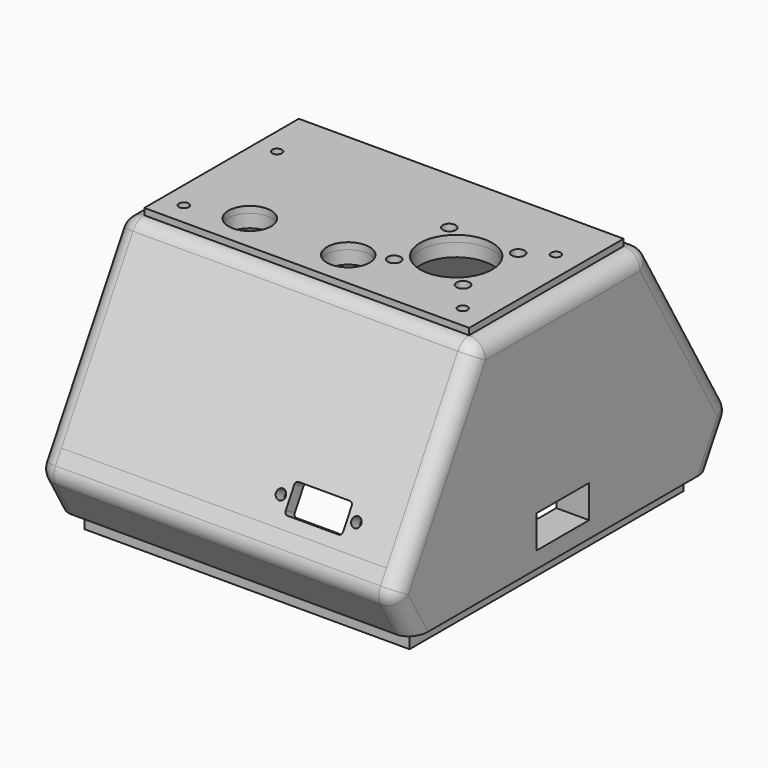
from build123d import *

# Parameters (mm, degrees)
F0_W          = 100
F0_H          = 60
F0_R          = 1.5
F0_R_2        = 6.5
F0_R_3        = 2
F0_R_4        = 11
F1_DEPTH      = 4
F2_R          = 2.5
F2_R_2        = 1.5
F3_DEPTH      = 35
F4_R          = 2.5
F4_R_2        = 1.5
F5_DEPTH      = 25
F6_W          = 2
F6_H          = 4
F7_DEPTH      = 100
F9_DEPTH      = 5
F10_W         = 30.2208131179
F10_H         = 20
F11_DEPTH     = 4
F13_DEPTH     = 109
F14_W         = 99
F14_H         = 104.2820323028
F15_DEPTH     = 6
F16_T1_DEPTH  = 58.8897274573
F16_T3_DEPTH  = 99
F16_T5_DEPTH  = 58.8452994616
F16_T7_DEPTH  = 24.6132486541
F16_T9_DEPTH  = 58.8897274573
F16_T11_DEPTH = 74.2764788033
F16_T13_DEPTH = 111.2168783649
F16_T15_DEPTH = 24.6132486541
F16_T17_DEPTH = 58.8897274573
F16_T22_DEPTH = 5
F16_T28_DEPTH = 5
F16_T34_DEPTH = 5
F16_T40_DEPTH = 5
F16_T46_DEPTH = 5
F16_T52_DEPTH = 5
F16_T58_DEPTH = 5
F17_W         = 89
F17_H         = 94.2820323028
F18_DEPTH     = 25
F19_W         = 20
F19_H         = 10
F20_DEPTH     = 10
F21_W         = 2
F21_H         = 2.6410161514
F21_W_2       = 3
F21_H_2       = 0.3589838486
F22_DEPTH     = 15
F23_R         = 1.25
F24_DEPTH     = 10
F25_R         = 0.99999
F26_W         = 17.5
F26_H         = 8.5
F26_R         = 1.5
F27_DEPTH     = 25
F28_R         = 1
F29_W         = 99
F29_H         = 58.8452994616
F29_R         = 1.5
F29_R_2       = 6.5
F29_R_3       = 2
F29_R_4       = 11
F30_DEPTH     = 2
F31_DEPTH     = 50


# Not quite as in the source:
# - a fillet or chamfer that OpenCascade refuses, or shapes differently, is made with other operations: its cross-section is extruded or revolved along the edge and cut away or added
# - a fillet or chamfer is up to 0.001 mm smaller than in the source, because OpenCascade refuses the exact size
# - a feature names something its author has since deleted; it is built from what else it names


with BuildPart() as f1:
    # F0 (on Top) → F1 (new body)
    with BuildSketch(Plane.XY):
        Rectangle(F0_W, F0_H)
        with Locations((-42.5, -22.5)):
            Circle(F0_R, mode=Mode.SUBTRACT)
        with Locations((-26, -18)):
            Circle(F0_R_2, mode=Mode.SUBTRACT)
        with Locations((4, -18)):
            Circle(F0_R_2, mode=Mode.SUBTRACT)
        with Locations((42.5, -22.5)):
            Circle(F0_R, mode=Mode.SUBTRACT)
        with Locations((14, -13)):
            Circle(F0_R_3, mode=Mode.SUBTRACT)
        with Locations((24.5, -2.5)):
            Circle(F0_R_4, mode=Mode.SUBTRACT)
        with Locations((35, -13)):
            Circle(F0_R_3, mode=Mode.SUBTRACT)
        with Locations((-42.5, 13)):
            Circle(F0_R, mode=Mode.SUBTRACT)
        with Locations((14, 8)):
            Circle(F0_R_3, mode=Mode.SUBTRACT)
        with Locations((35, 8)):
            Circle(F0_R_3, mode=Mode.SUBTRACT)
        with Locations((42.5, 13)):
            Circle(F0_R, mode=Mode.SUBTRACT)
    extrude(amount=F1_DEPTH)

    # F2 (on face) → F3 (join)
    with BuildSketch(Plane(origin=(0, 0, 0), x_dir=(1, 0, 0), z_dir=(0, 0, -1))):
        with Locations((-42.5, 22.5)):
            Circle(F2_R)
        with Locations((-42.5, 22.5)):
            Circle(F2_R_2, mode=Mode.SUBTRACT)
        with Locations((-42.5, -13)):
            Circle(F2_R)
        with Locations((-42.5, -13)):
            Circle(F2_R_2, mode=Mode.SUBTRACT)
        with Locations((42.5, -13)):
            Circle(F2_R)
        with Locations((42.5, -13)):
            Circle(F2_R_2, mode=Mode.SUBTRACT)
        with Locations((42.5, 22.5)):
            Circle(F2_R)
        with Locations((42.5, 22.5)):
            Circle(F2_R_2, mode=Mode.SUBTRACT)
    extrude(amount=F3_DEPTH)

    # F4 (on face) → F5 (join)
    with BuildSketch(Plane.XY.offset(4)):
        with Locations((-42.5, 13)):
            Circle(F4_R)
        with Locations((-42.5, 13)):
            Circle(F4_R_2, mode=Mode.SUBTRACT)
        with Locations((42.5, 13)):
            Circle(F4_R_2)
        with Locations((42.5, -22.5)):
            Circle(F4_R_2)
        with Locations((-42.5, -22.5)):
            Circle(F4_R)
        with Locations((-42.5, -22.5)):
            Circle(F4_R_2, mode=Mode.SUBTRACT)
    extrude(amount=-F5_DEPTH)

    # F6 (on face) → F7 (join)
    with BuildSketch(Plane.YZ.offset(50)):
        with Locations((-29, 2)):
            Rectangle(F6_W, F6_H)
        Polygon((-57.5, -47.6313972081), (-30, 0), (-30, 4), (-32.3094010768, 4), (-33.4641016151, 2), (-60.9641016151, -45.6313972081), (-64.6410161514, -52), (-60.0222139979, -52), align=None)
        with Locations((29, 2)):
            Rectangle(F6_W, F6_H)
        Polygon((30, 4), (30, 0), (57.5, -47.6313972081), (60.0222139979, -52), (64.6410161514, -52), (60.9641016151, -45.6313972081), (33.4641016151, 2), (32.3094010768, 4), align=None)
    extrude(amount=-F7_DEPTH)

    # F8 (on face) → F9 (join)
    with BuildSketch(Plane.YZ.offset(50)):
        Polygon((-32.3094010768, 4), (-64.6410161514, -52), (64.6410161514, -52), (32.3094010768, 4), align=None)
    extrude(amount=F9_DEPTH)

    # F10 (on face) → F11 (join)
    with BuildSketch(Plane(origin=(-50, 0, 0), x_dir=(0, -1, 0), z_dir=(-1, 0, 0))):
        Polygon((-32.3094010768, 4), (-64.6410161514, -52), (64.6410161514, -52), (32.3094010768, 4), align=None)
        with Locations((4.7969543375, -25.0177697837)):
            Rectangle(F10_W, F10_H, mode=Mode.SUBTRACT)
    extrude(amount=F11_DEPTH)

    # F12 (on face) → F13 (join, through all)
    with BuildSketch(Plane(origin=(-54, 0, 0), x_dir=(0, -1, 0), z_dir=(-1, 0, 0))):
        Polygon((-63.0000010133, -52), (-64.6410161514, -52), (-57.1410161514, -64.9903810568), (57.1410161514, -64.9903810568), (64.6410161514, -52), align=None)
    extrude(amount=-F13_DEPTH)

    # F14 (on face) → F15 (join)
    with BuildSketch(Plane(origin=(0, 0, -64.9903810568), x_dir=(1, 0, 0), z_dir=(0, 0, -1))):
        with Locations((0.5, 0)):
            Rectangle(F14_W, F14_H)
    extrude(amount=F15_DEPTH)

    # F16: fillet of radius 5 on 13 edges, made by hand

    # F16_s2 → F16_t1 (cut)
    with BuildSketch(Plane(origin=(0, -37.2335388633, -64.4903810568), x_dir=(1, 0, 0), z_dir=(0, 0.5, 0.8660254038))):
        with BuildLine():
            ThreePointArc((-54, -24.9807621135), (-52.5355339059, -28.5162960195), (-49, -29.9807621135))
            Line((-49, -29.9807621135), (-54, -29.9807621135))
            Line((-54, -29.9807621135), (-54, -24.9807621135))
        make_face()
    extrude(amount=F16_T1_DEPTH, mode=Mode.SUBTRACT)

    # F16_s4 → F16_t3 (cut)
    with BuildSketch(Plane.YZ.offset(-49)):
        with BuildLine():
            ThreePointArc((-29.4226497308, 4), (-31.9226497308, 3.3301270189), (-33.7527767497, 1.5))
            Line((-33.7527767497, 1.5), (-32.3094010768, 4))
            Line((-32.3094010768, 4), (-29.4226497308, 4))
        make_face()
        with BuildLine():
            ThreePointArc((-63.1976404784, -49.5), (-63.8675134595, -52), (-63.1976404784, -54.5))
            Line((-63.1976404784, -54.5), (-64.6410161514, -52))
            Line((-64.6410161514, -52), (-63.1976404784, -49.5))
        make_face()
        with BuildLine():
            ThreePointArc((29.4226497308, 4), (31.9226497308, 3.3301270189), (33.7527767497, 1.5))
            Line((33.7527767497, 1.5), (32.3094010768, 4))
            Line((32.3094010768, 4), (29.4226497308, 4))
        make_face()
    extrude(amount=F16_T3_DEPTH, mode=Mode.SUBTRACT)

    # F16_s6 → F16_t5 (cut)
    with BuildSketch(Plane.XZ.offset(-29.4226497308)):
        with BuildLine():
            ThreePointArc((-49, 4), (-52.5355339059, 2.5355339059), (-54, -1))
            Line((-54, -1), (-54, 4))
            Line((-54, 4), (-49, 4))
        make_face()
        with BuildLine():
            ThreePointArc((50, 4), (53.5355339059, 2.5355339059), (55, -1))
            Line((55, -1), (55, 4))
            Line((55, 4), (50, 4))
        make_face()
    extrude(amount=F16_T5_DEPTH, mode=Mode.SUBTRACT)

    # F16_s8 → F16_t7 (cut)
    with BuildSketch(Plane(origin=(0, 20.1064064606, -34.8253175473), x_dir=(1, 0, 0), z_dir=(0, -0.5, 0.8660254038))):
        with BuildLine():
            ThreePointArc((-54, -76.9807621135), (-52.5355339059, -80.5162960195), (-49, -81.9807621135))
            Line((-49, -81.9807621135), (-54, -81.9807621135))
            Line((-54, -81.9807621135), (-54, -76.9807621135))
        make_face()
        with BuildLine():
            ThreePointArc((55, -76.9807621135), (53.5355339059, -80.5162960195), (50, -81.9807621135))
            Line((50, -81.9807621135), (55, -81.9807621135))
            Line((55, -81.9807621135), (55, -76.9807621135))
        make_face()
    extrude(amount=F16_T7_DEPTH, mode=Mode.SUBTRACT)

    # F16_s10 → F16_t9 (cut)
    with BuildSketch(Plane(origin=(0, -7.7886751346, -13.4903810568), x_dir=(1, 0, 0), z_dir=(0, -0.5, -0.8660254038))):
        with BuildLine():
            ThreePointArc((50, 29.9807621135), (53.5355339059, 28.5162960195), (55, 24.9807621135))
            Line((55, 24.9807621135), (55, 29.9807621135))
            Line((55, 29.9807621135), (50, 29.9807621135))
        make_face()
    extrude(amount=F16_T9_DEPTH, mode=Mode.SUBTRACT)

    # F16_s12 → F16_t11 (cut)
    with BuildSketch(Plane(origin=(0, 7.7886751346, -13.4903810568), x_dir=(1, 0, 0), z_dir=(0, 0.5, -0.8660254038))):
        with BuildLine():
            ThreePointArc((-54, -24.9807621135), (-52.5355339059, -28.5162960195), (-49, -29.9807621135))
            Line((-49, -29.9807621135), (-54, -29.9807621135))
            Line((-54, -29.9807621135), (-54, -24.9807621135))
        make_face()
    extrude(amount=F16_T11_DEPTH, mode=Mode.SUBTRACT)

    # F16_s14 → F16_t13 (cut)
    with BuildSketch(Plane.YZ.offset(-61.2168783649)):
        with BuildLine():
            ThreePointArc((63.1976404784, -49.5), (63.8675134595, -52), (63.1976404784, -54.5))
            Line((63.1976404784, -54.5), (64.6410161514, -52))
            Line((64.6410161514, -52), (63.1976404784, -49.5))
        make_face()
    extrude(amount=F16_T13_DEPTH, mode=Mode.SUBTRACT)

    # F16_s16 → F16_t15 (cut)
    with BuildSketch(Plane(origin=(0, -7.7997821335, -13.5096189432), x_dir=(1, 0, 0), z_dir=(0, -0.5, -0.8660254038))):
        with BuildLine():
            ThreePointArc((55, -76.9807621135), (53.5355339059, -80.5162960195), (50, -81.9807621135))
            Line((50, -81.9807621135), (55, -81.9807621135))
            Line((55, -81.9807621135), (55, -76.9807621135))
        make_face()
    extrude(amount=F16_T15_DEPTH, mode=Mode.SUBTRACT)

    # F16_s18 → F16_t17 (cut)
    with BuildSketch(Plane(origin=(0, 37.2335388633, -64.4903810568), x_dir=(1, 0, 0), z_dir=(0, -0.5, 0.8660254038))):
        with BuildLine():
            ThreePointArc((50, 29.9807621135), (53.5355339059, 28.5162960195), (55, 24.9807621135))
            Line((55, 24.9807621135), (55, 29.9807621135))
            Line((55, 29.9807621135), (50, 29.9807621135))
        make_face()
    extrude(amount=F16_T17_DEPTH, mode=Mode.SUBTRACT)


with BuildPart() as f16_tool20:
    # F16_s21 → F16_t22 (new body)
    with BuildSketch(Plane.YZ.offset(-49)):
        Polygon((-58.8675134595, -52), (-63.1976404784, -54.5), (-64.6410161514, -52), (-63.1976404784, -49.5), align=None)
    extrude(amount=-F16_T22_DEPTH)

    # F16_s23 → F16_t24 (revolve, cut)
    with BuildSketch(Plane(origin=(-49, -58.8675134595, -52), x_dir=(0, 1, 0), z_dir=(0, 0, 1))):
        with BuildLine():
            ThreePointArc((0, -5), (5, 0), (0, 5))
            Line((0, 5), (0, -5))
        make_face()
    revolve(axis=Axis((-49, -58.8675134595, -52), (-1, 0, 0)), mode=Mode.SUBTRACT)


with BuildPart() as f1_1:
    add(f1.part)

    # F16_t19: cut F16_tool20
    add(f16_tool20.part, mode=Mode.SUBTRACT)


with BuildPart() as f16_tool26:
    # F16_s27 → F16_t28 (new body)
    with BuildSketch(Plane.YZ.offset(-49)):
        Polygon((-29.4226497308, -1), (-33.7527767497, 1.5), (-32.3094010768, 4), (-29.4226497308, 4), align=None)
    extrude(amount=-F16_T28_DEPTH)

    # F16_s29 → F16_t30 (revolve, cut)
    with BuildSketch(Plane(origin=(-49, -29.4226497308, -1), x_dir=(0, 0.5, -0.8660254038), z_dir=(0, 0.8660254038, 0.5))):
        with BuildLine():
            ThreePointArc((0, -5), (5, 0), (0, 5))
            Line((0, 5), (0, -5))
        make_face()
    revolve(axis=Axis((-49, -29.4226497308, -1), (-1, 0, 0)), mode=Mode.SUBTRACT)


with BuildPart() as f1_2:
    add(f1_1.part)

    # F16_t25: cut F16_tool26
    add(f16_tool26.part, mode=Mode.SUBTRACT)


with BuildPart() as f16_tool32:
    # F16_s33 → F16_t34 (new body)
    with BuildSketch(Plane.YZ.offset(50)):
        Polygon((-29.4226497308, -1), (-33.7527767497, 1.5), (-32.3094010768, 4), (-29.4226497308, 4), align=None)
    extrude(amount=F16_T34_DEPTH)

    # F16_s35 → F16_t36 (revolve, cut)
    with BuildSketch(Plane(origin=(50, -29.4226497308, -1), x_dir=(0, 0.5, -0.8660254038), z_dir=(0, -0.8660254038, -0.5))):
        with BuildLine():
            ThreePointArc((0, -5), (5, 0), (0, 5))
            Line((0, 5), (0, -5))
        make_face()
    revolve(axis=Axis((50, -29.4226497308, -1), (1, 0, 0)), mode=Mode.SUBTRACT)


with BuildPart() as f1_3:
    add(f1_2.part)

    # F16_t31: cut F16_tool32
    add(f16_tool32.part, mode=Mode.SUBTRACT)


with BuildPart() as f16_tool38:
    # F16_s39 → F16_t40 (new body)
    with BuildSketch(Plane.YZ.offset(-49)):
        Polygon((29.4226497308, -1), (33.7527767497, 1.5), (32.3094010768, 4), (29.4226497308, 4), align=None)
    extrude(amount=-F16_T40_DEPTH)

    # F16_s41 → F16_t42 (revolve, cut)
    with BuildSketch(Plane(origin=(-49, 29.4226497308, -1), x_dir=(0, -0.5, -0.8660254038), z_dir=(0, 0.8660254038, -0.5))):
        with BuildLine():
            ThreePointArc((0, -5), (5, 0), (0, 5))
            Line((0, 5), (0, -5))
        make_face()
    revolve(axis=Axis((-49, 29.4226497308, -1), (-1, 0, 0)), mode=Mode.SUBTRACT)


with BuildPart() as f1_4:
    add(f1_3.part)

    # F16_t37: cut F16_tool38
    add(f16_tool38.part, mode=Mode.SUBTRACT)


with BuildPart() as f16_tool44:
    # F16_s45 → F16_t46 (new body)
    with BuildSketch(Plane.YZ.offset(50)):
        Polygon((-58.8675134595, -52), (-63.1976404784, -54.5), (-64.6410161514, -52), (-63.1976404784, -49.5), align=None)
    extrude(amount=F16_T46_DEPTH)

    # F16_s47 → F16_t48 (revolve, cut)
    with BuildSketch(Plane(origin=(50, -58.8675134595, -52), x_dir=(0, 1, 0), z_dir=(0, 0, -1))):
        with BuildLine():
            ThreePointArc((0, -5), (5, 0), (0, 5))
            Line((0, 5), (0, -5))
        make_face()
    revolve(axis=Axis((50, -58.8675134595, -52), (1, 0, 0)), mode=Mode.SUBTRACT)


with BuildPart() as f1_5:
    add(f1_4.part)

    # F16_t43: cut F16_tool44
    add(f16_tool44.part, mode=Mode.SUBTRACT)


with BuildPart() as f16_tool50:
    # F16_s51 → F16_t52 (new body)
    with BuildSketch(Plane.YZ.offset(50)):
        Polygon((29.4226497308, -1), (33.7527767497, 1.5), (32.3094010768, 4), (29.4226497308, 4), align=None)
    extrude(amount=F16_T52_DEPTH)

    # F16_s53 → F16_t54 (revolve, cut)
    with BuildSketch(Plane(origin=(50, 29.4226497308, -1), x_dir=(0, -0.5, -0.8660254038), z_dir=(0, -0.8660254038, 0.5))):
        with BuildLine():
            ThreePointArc((0, -5), (5, 0), (0, 5))
            Line((0, 5), (0, -5))
        make_face()
    revolve(axis=Axis((50, 29.4226497308, -1), (1, 0, 0)), mode=Mode.SUBTRACT)


with BuildPart() as f1_6:
    add(f1_5.part)

    # F16_t49: cut F16_tool50
    add(f16_tool50.part, mode=Mode.SUBTRACT)


with BuildPart() as f16_tool56:
    # F16_s57 → F16_t58 (new body)
    with BuildSketch(Plane.YZ.offset(50)):
        Polygon((58.8675134595, -52), (63.1976404784, -54.5), (64.6410161514, -52), (63.1976404784, -49.5), align=None)
    extrude(amount=F16_T58_DEPTH)

    # F16_s59 → F16_t60 (revolve, cut)
    with BuildSketch(Plane(origin=(50, 58.8675134595, -52), x_dir=(0, -1, 0), z_dir=(0, 0, 1))):
        with BuildLine():
            ThreePointArc((0, -5), (5, 0), (0, 5))
            Line((0, 5), (0, -5))
        make_face()
    revolve(axis=Axis((50, 58.8675134595, -52), (1, 0, 0)), mode=Mode.SUBTRACT)


with BuildPart() as f1_7:
    add(f1_6.part)

    # F16_t55: cut F16_tool56
    add(f16_tool56.part, mode=Mode.SUBTRACT)

    # F17 (on face) → F18 (cut)
    with BuildSketch(Plane(origin=(0, 0, -70.9903810568), x_dir=(1, 0, 0), z_dir=(0, 0, -1))):
        with Locations((0.5, 0)):
            Rectangle(F17_W, F17_H)
    extrude(amount=-F18_DEPTH, mode=Mode.SUBTRACT)

    # F19 (on face) → F20 (cut)
    with BuildSketch(Plane.YZ.offset(55)):
        with Locations((0, -54.9903810568)):
            Rectangle(F19_W, F19_H)
    extrude(amount=-F20_DEPTH, mode=Mode.SUBTRACT)

    # F21 (on face) → F22 (join)
    with BuildSketch(Plane(origin=(0, 0, -70.9903810568), x_dir=(1, 0, 0), z_dir=(0, 0, -1))):
        Polygon((-42, -47.5), (-45, -47.5), (-45, -44.5), (-48, -44.5), (-48, -50.5), (-42, -50.5), align=None)
        with Locations((-43, -45.8205080757)):
            Rectangle(F21_W, F21_H)
        Polygon((-45, -44.5), (-45, -47.5), (-42, -47.5), (-42, -47.1410161514), (-44, -47.1410161514), (-44, -44.5), align=None)
        with Locations((43.5, -45.8205080757)):
            Rectangle(F21_W_2, F21_H)
        Polygon((45, -47.5), (42, -47.5), (42, -50.5), (48, -50.5), (48, -44.5), (45, -44.5), (45, -47.1410161514), align=None)
        with Locations((43.5, -47.3205080757)):
            Rectangle(F21_W_2, F21_H_2)
        with Locations((43.5, 47.3205080757)):
            Rectangle(F21_W_2, F21_H_2)
        with Locations((43.5, 45.8205080757)):
            Rectangle(F21_W_2, F21_H)
        Polygon((42, 50.5), (42, 47.5), (45, 47.5), (45, 47.1410161514), (45, 44.5), (48, 44.5), (48, 50.5), align=None)
        with Locations((-43, 45.8205080757)):
            Rectangle(F21_W, F21_H)
        Polygon((-45, 47.5), (-45, 44.5), (-44, 44.5), (-44, 47.1410161514), (-42, 47.1410161514), (-42, 47.5), align=None)
        Polygon((-48, 44.5), (-45, 44.5), (-45, 47.5), (-42, 47.5), (-42, 50.5), (-48, 50.5), align=None)
    extrude(amount=-F22_DEPTH)

    # F23 (on face) → F24 (cut)
    with BuildSketch(Plane(origin=(0, 0, -70.9903810568), x_dir=(1, 0, 0), z_dir=(0, 0, -1))):
        with Locations((-45, 47.5)):
            Circle(F23_R)
        with Locations((45, 47.5)):
            Circle(F23_R)
        with Locations((45, -47.5)):
            Circle(F23_R)
        with Locations((-45, -47.5)):
            Circle(F23_R)
    extrude(amount=-F24_DEPTH, mode=Mode.SUBTRACT)

    # F25 (radius 1 in the source; OpenCascade refuses exactly that, so slightly less here)
    f25_edges = [f1_7.edges().sort_by_distance(p)[0] for p in [
        (45, 44.5, -63.490381),
        (42, 44.5, -63.490381),
        (42, 47.141016, -63.490381),
        (-42, 47.141016, -63.490381),
        (-42, 44.5, -63.490381),
        (-44, 44.5, -63.490381),
        (-44, -44.5, -63.490381),
        (-42, -44.5, -63.490381),
        (-42, -47.141016, -63.490381),
        (45, -44.5, -63.490381),
        (42, -44.5, -63.490381),
        (42, -47.141016, -63.490381),
    ]]
    fillet(f25_edges, radius=F25_R)

    # F26 (on face) → F27 (cut)
    with BuildSketch(Plane(origin=(0, -25.9641016151, 14.9903810568), x_dir=(1, 0, 0), z_dir=(0, -0.8660254038, 0.5))):
        with Locations((26.25, -62.2170777265)):
            Rectangle(F26_W, F26_H)
        with Locations((37.75, -62.2170777265)):
            Circle(F26_R)
        with Locations((14.75, -62.2170777265)):
            Circle(F26_R)
    extrude(amount=-F27_DEPTH, mode=Mode.SUBTRACT)

    # F28
    f28_edges = [f1_7.edges().sort_by_distance(p)[0] for p in [
        (17.5, -53.21559, -36.210581),
        (35, -53.21559, -36.210581),
        (17.5, -57.46559, -43.571797),
        (35, -57.46559, -43.571797),
    ]]
    fillet(f28_edges, radius=F28_R)


with BuildPart() as f30:
    # F29 (on face) → F30 (new body)
    with BuildSketch(Plane.XY.offset(4)):
        with Locations((0.5, 0)):
            Rectangle(F29_W, F29_H)
        with Locations((-42.5, -22.5)):
            Circle(F29_R, mode=Mode.SUBTRACT)
        with Locations((-26, -18)):
            Circle(F29_R_2, mode=Mode.SUBTRACT)
        with Locations((4, -18)):
            Circle(F29_R_2, mode=Mode.SUBTRACT)
        with BuildLine():
            ThreePointArc((34.3146883861, 4.5677488449), (36.0105746079, 1.2131999738), (36.5946757646, -2.5))
            ThreePointArc((36.5946757646, -2.5), (36.0105746079, -6.2131999738), (34.3146883861, -9.5677488449))
            ThreePointArc((34.3146883861, -9.5677488449), (37.2193928619, -10.2936564659), (38.5, -13))
            ThreePointArc((38.5, -13), (34.6556738776, -16.483021608), (31.5677488449, -12.3146883861))
            ThreePointArc((31.5677488449, -12.3146883861), (24.5, -14.5946757646), (17.4322511551, -12.3146883861))
            ThreePointArc((17.4322511551, -12.3146883861), (17.483021608, -12.6556738776), (17.5, -13))
            ThreePointArc((17.5, -13), (11.2936564659, -15.2193928619), (14.6853116139, -9.5677488449))
            ThreePointArc((14.6853116139, -9.5677488449), (12.4053242354, -2.5), (14.6853116139, 4.5677488449))
            ThreePointArc((14.6853116139, 4.5677488449), (11.2936564659, 10.2193928619), (17.5, 8))
            ThreePointArc((17.5, 8), (17.483021608, 7.6556738776), (17.4322511551, 7.3146883861))
            ThreePointArc((17.4322511551, 7.3146883861), (24.5, 9.5946757646), (31.5677488449, 7.3146883861))
            ThreePointArc((31.5677488449, 7.3146883861), (34.6556738776, 11.483021608), (38.5, 8))
            ThreePointArc((38.5, 8), (37.2193928619, 5.2936564659), (34.3146883861, 4.5677488449))
        make_face(mode=Mode.SUBTRACT)
        with Locations((-42.5, 13)):
            Circle(F29_R, mode=Mode.SUBTRACT)
        with BuildLine():
            ThreePointArc((14.6853116139, 4.5677488449), (15.9477727506, 6.0522272494), (17.4322511551, 7.3146883861))
            ThreePointArc((17.4322511551, 7.3146883861), (17.483021608, 7.6556738776), (17.5, 8))
            ThreePointArc((17.5, 8), (11.2936564659, 10.2193928619), (14.6853116139, 4.5677488449))
        make_face()
        with Locations((14, 8)):
            Circle(F29_R_3, mode=Mode.SUBTRACT)
        with BuildLine():
            ThreePointArc((31.5677488449, 7.3146883861), (33.0522272494, 6.0522272494), (34.3146883861, 4.5677488449))
            ThreePointArc((34.3146883861, 4.5677488449), (37.2193928619, 5.2936564659), (38.5, 8))
            ThreePointArc((38.5, 8), (34.6556738776, 11.483021608), (31.5677488449, 7.3146883861))
        make_face()
        with Locations((35, 8)):
            Circle(F29_R_3, mode=Mode.SUBTRACT)
        with BuildLine():
            ThreePointArc((38.5, -13), (37.2193928619, -10.2936564659), (34.3146883861, -9.5677488449))
            ThreePointArc((34.3146883861, -9.5677488449), (33.0522272494, -11.0522272494), (31.5677488449, -12.3146883861))
            ThreePointArc((31.5677488449, -12.3146883861), (34.6556738776, -16.483021608), (38.5, -13))
        make_face()
        with Locations((35, -13)):
            Circle(F29_R_3, mode=Mode.SUBTRACT)
        with BuildLine():
            ThreePointArc((17.5, -13), (17.483021608, -12.6556738776), (17.4322511551, -12.3146883861))
            ThreePointArc((17.4322511551, -12.3146883861), (15.9477727506, -11.0522272494), (14.6853116139, -9.5677488449))
            ThreePointArc((14.6853116139, -9.5677488449), (11.2936564659, -15.2193928619), (17.5, -13))
        make_face()
        with Locations((14, -13)):
            Circle(F29_R_3, mode=Mode.SUBTRACT)
        with BuildLine():
            ThreePointArc((34.3146883861, -9.5677488449), (36.0105746079, -6.2131999738), (36.5946757646, -2.5))
            ThreePointArc((36.5946757646, -2.5), (36.0105746079, 1.2131999738), (34.3146883861, 4.5677488449))
            ThreePointArc((34.3146883861, 4.5677488449), (32.5251262658, 5.5251262658), (31.5677488449, 7.3146883861))
            ThreePointArc((31.5677488449, 7.3146883861), (24.5, 9.5946757646), (17.4322511551, 7.3146883861))
            ThreePointArc((17.4322511551, 7.3146883861), (16.4748737342, 5.5251262658), (14.6853116139, 4.5677488449))
            ThreePointArc((14.6853116139, 4.5677488449), (12.4053242354, -2.5), (14.6853116139, -9.5677488449))
            ThreePointArc((14.6853116139, -9.5677488449), (16.4748737342, -10.5251262658), (17.4322511551, -12.3146883861))
            ThreePointArc((17.4322511551, -12.3146883861), (24.5, -14.5946757646), (31.5677488449, -12.3146883861))
            ThreePointArc((31.5677488449, -12.3146883861), (32.5251262658, -10.5251262658), (34.3146883861, -9.5677488449))
        make_face()
        with Locations((24.5, -2.5)):
            Circle(F29_R_4, mode=Mode.SUBTRACT)
        with BuildLine():
            ThreePointArc((31.5677488449, 7.3146883861), (32.5251262658, 5.5251262658), (34.3146883861, 4.5677488449))
            ThreePointArc((34.3146883861, 4.5677488449), (33.0522272494, 6.0522272494), (31.5677488449, 7.3146883861))
        make_face()
        with BuildLine():
            ThreePointArc((14.6853116139, 4.5677488449), (16.4748737342, 5.5251262658), (17.4322511551, 7.3146883861))
            ThreePointArc((17.4322511551, 7.3146883861), (15.9477727506, 6.0522272494), (14.6853116139, 4.5677488449))
        make_face()
        with BuildLine():
            ThreePointArc((14.6853116139, -9.5677488449), (15.9477727506, -11.0522272494), (17.4322511551, -12.3146883861))
            ThreePointArc((17.4322511551, -12.3146883861), (16.4748737342, -10.5251262658), (14.6853116139, -9.5677488449))
        make_face()
        with BuildLine():
            ThreePointArc((31.5677488449, -12.3146883861), (33.0522272494, -11.0522272494), (34.3146883861, -9.5677488449))
            ThreePointArc((34.3146883861, -9.5677488449), (32.5251262658, -10.5251262658), (31.5677488449, -12.3146883861))
        make_face()
    extrude(amount=F30_DEPTH)


with BuildPart() as f31_tool:
    # F31 (cut): faces of the model
    f31_faces = [f1_7.part.faces().sort_by_distance(p)[0] for p in [
        (42.5, 13, -21),
        (42.5, -22.5, -21),
    ]]
    extrude(f31_faces, amount=-F31_DEPTH)


with BuildPart() as f1_8:
    add(f1_7.part)

    # F31: cut by f31_tool
    add(f31_tool.part, mode=Mode.SUBTRACT)


with BuildPart() as f30_1:
    add(f30.part)

    # F31: cut by f31_tool
    add(f31_tool.part, mode=Mode.SUBTRACT)


solid = Compound([f1_8.part, f30_1.part])
